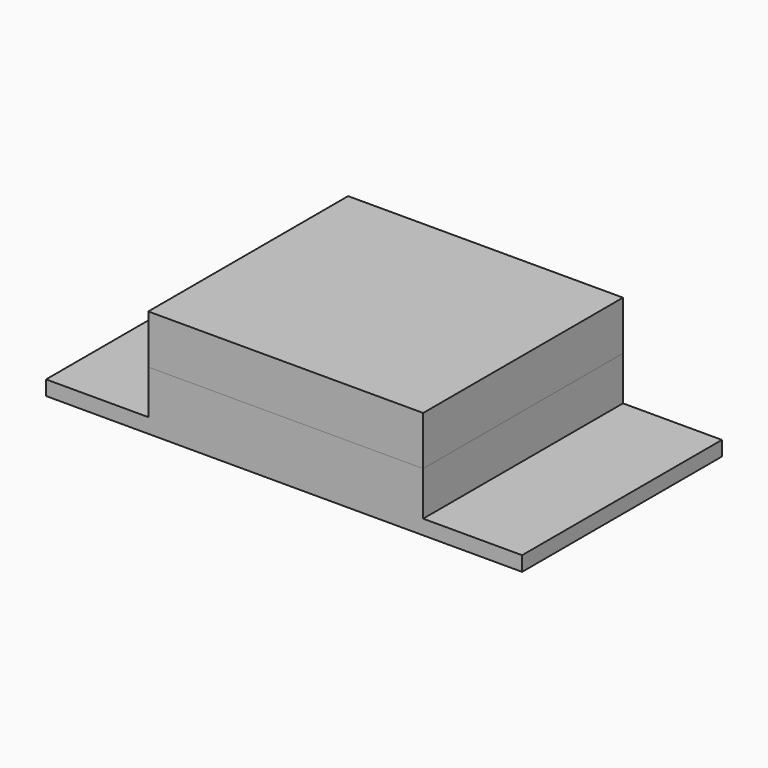
from build123d import *

# Parameters (mm, degrees)
F0_W     = 9.1
F0_H     = 23.5
F1_DEPTH = 1.5
F0_W_2   = 9.4355237663
F0_W_3   = 27.0644762337
F0_H_2   = 24.5
F2_DEPTH = 6
F0_W_4   = 12.3644762337
F0_H_3   = 11.25
F0_W_5   = 12.7
F3_DEPTH = 10
F4_W     = 28.0644762337
F4_H     = 25.5
F4_W_2   = 27.0644762337
F4_H_2   = 24.5
F5_DEPTH = 4
F6_W     = 28.0644762337
F6_H     = 25.5
F7_DEPTH = 1


with BuildPart() as f1:
    # F0 (on Top) → F1 (new body)
    with BuildSketch(Plane.XY):
        with Locations((18.75, 0)):
            Rectangle(F0_W, F0_H)
        Polygon((24.3, -12.75), (24.3, 12.75), (14.2, 12.75), (14.2, 11.75), (23.3, 11.75), (23.3, -11.75), (14.2, -11.75), (14.2, -12.75), align=None)
    extrude(amount=F1_DEPTH)



with BuildPart() as f1b:
    # F0 (on Top) → F1, piece 2 (new body)
    with BuildSketch(Plane.XY):
        Polygon((-13.8644762337, 11.75), (-13.8644762337, 12.75), (-24.3, 12.75), (-24.3, -12.75), (-13.8644762337, -12.75), (-13.8644762337, -11.75), (-23.3, -11.75), (-23.3, 11.75), align=None)
        with Locations((-18.5822381169, 0)):
            Rectangle(F0_W_2, F0_H)
    extrude(amount=F1_DEPTH)


with BuildPart() as f1_1:
    add(f1.part)

    add(f1b.part)  # F2 merges F1b
    # F0 (on Top) → F2 (join)
    with BuildSketch(Plane.XY):
        Polygon((14.2, 11.75), (14.2, 12.75), (-13.8644762337, 12.75), (-13.8644762337, 11.75), (-13.8644762337, -11.75), (-13.8644762337, -12.75), (14.2, -12.75), (14.2, -11.75), align=None)
        with Locations((0.1677618831, 0)):
            Rectangle(F0_W_3, F0_H_2, mode=Mode.SUBTRACT)
    extrude(amount=F2_DEPTH)

    # F0 (on Top) → F3 (join)
    with BuildSketch(Plane.XY):
        with Locations((0.1677618831, 0)):
            Rectangle(F0_W_3, F0_H_2)
        with Locations((-6.6822381169, -6.125)):
            Rectangle(F0_W_4, F0_H_3, mode=Mode.SUBTRACT)
        with Locations((6.85, -6.125)):
            Rectangle(F0_W_5, F0_H_3, mode=Mode.SUBTRACT)
        with Locations((-6.6822381169, 6.125)):
            Rectangle(F0_W_4, F0_H_3, mode=Mode.SUBTRACT)
        with Locations((6.85, 6.125)):
            Rectangle(F0_W_5, F0_H_3, mode=Mode.SUBTRACT)
    extrude(amount=F3_DEPTH)


with BuildPart() as f5:
    # F4 (on face) → F5 (new body)
    with BuildSketch(Plane.XY.offset(6)):
        with Locations((0.1677618831, 0)):
            Rectangle(F4_W, F4_H)
        with Locations((0.1677618831, 0)):
            Rectangle(F4_W_2, F4_H_2, mode=Mode.SUBTRACT)
    extrude(amount=F5_DEPTH)

    # F6 (on face) → F7 (join)
    with BuildSketch(Plane.XY.offset(10)):
        with Locations((0.1677618831, 0)):
            Rectangle(F6_W, F6_H)
    extrude(amount=F7_DEPTH)


solid = Compound([f1_1.part, f5.part])
